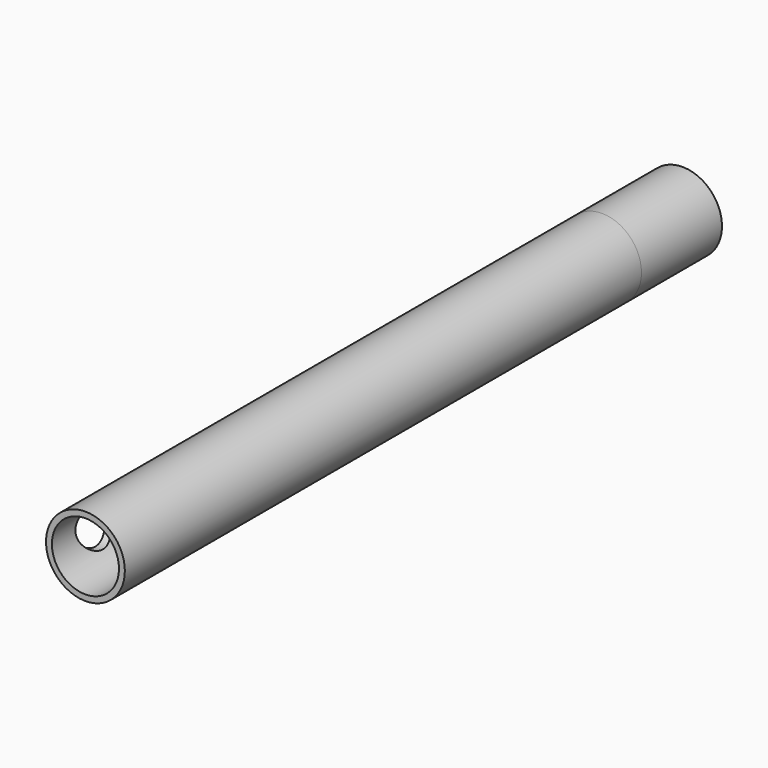
from build123d import *

# Parameters (mm, degrees)
F3_R      = 4.7
F4_DEPTH  = 67
F8_DEPTH  = 67
F6_R      = 4.7
F6_R_2    = 4
F9_DEPTH  = 10
F7_R      = 4.7
F7_R_2    = 4
F10_DEPTH = 12
F11_R     = 2.75
F12_DEPTH = 4.701


# Not quite as in the source:
# - ends of sketch curves that miss each other by under 0.0002 mm in the source are joined


with BuildPart() as f4:
    # F3 (on Front) → F4 (new body)
    with BuildSketch(Plane.XZ):
        Circle(F3_R)
    extrude(amount=F4_DEPTH)

    # F5 (on face) → F8 (cut, through all)
    with BuildSketch(Plane.XZ.offset(67)):
        with BuildLine():
            Line((-1.25, -3.8), (0, -3.8))
            Line((0, -3.8), (1.25, -3.8))
            Line((1.25, -3.8), (1.25, -3.7))
            ThreePointArc((1.25, -3.7), (1.3085786438, -3.5585786438), (1.45, -3.5))
            Line((1.45, -3.5), (2, -3.5))
            Line((2, -3.5), (2, -3.05))
            ThreePointArc((2, -3.05), (2.0585786438, -2.9085786438), (2.2, -2.85))
            Line((2.2, -2.85), (3.15, -2.85))
            Line((3.15, -2.85), (3.15, -2.15))
            Line((3.15, -2.15), (2.2, -2.15))
            ThreePointArc((2.2, -2.15), (2.0585786438, -2.0914213562), (2, -1.95))
            Line((2, -1.95), (2, -1.887459))
            ThreePointArc((2, -1.887459), (2.1033535752, -1.771554046), (2.2, -1.65))
            Line((2.2, -1.65), (3.75, -1.65))
            Line((3.75, -1.65), (3.75, 0))
            Line((3.75, 0), (3.75, 1.65))
            Line((3.75, 1.65), (2.2, 1.65))
            ThreePointArc((2.2, 1.65), (2.1033535752, 1.771554046), (1.9999998047, 1.8874588157))
            Line((1.9999998047, 1.8874588157), (2, 1.95))
            ThreePointArc((2, 1.95), (2.0585786438, 2.0914213562), (2.2, 2.15))
            Line((2.2, 2.15), (3.15, 2.15))
            Line((3.15, 2.15), (3.15, 2.85))
            Line((3.15, 2.85), (2.2, 2.85))
            ThreePointArc((2.2, 2.85), (2.0585786438, 2.9085786438), (2, 3.05))
            Line((2, 3.05), (2, 3.5))
            Line((2, 3.5), (1.45, 3.5))
            ThreePointArc((1.45, 3.5), (1.3085786438, 3.5585786438), (1.25, 3.7))
            Line((1.25, 3.7), (1.25, 3.8))
            Line((1.25, 3.8), (0, 3.8))
            Line((0, 3.8), (-1.25, 3.8))
            Line((-1.25, 3.8), (-1.25, 3.7))
            ThreePointArc((-1.25, 3.7), (-1.3085786438, 3.5585786438), (-1.45, 3.5))
            Line((-1.45, 3.5), (-2, 3.5))
            Line((-2, 3.5), (-2, 3.05))
            ThreePointArc((-2, 3.05), (-2.0585786438, 2.9085786438), (-2.2, 2.85))
            Line((-2.2, 2.85), (-3.15, 2.85))
            Line((-3.15, 2.85), (-3.15, 2.15))
            Line((-3.15, 2.15), (-2.2, 2.15))
            ThreePointArc((-2.2, 2.15), (-2.0585786438, 2.0914213562), (-2, 1.95))
            Line((-2, 1.95), (-2, 1.887459))
            ThreePointArc((-2, 1.887459), (-2.1033535752, 1.771554046), (-2.2, 1.65))
            Line((-2.2, 1.65), (-3.75, 1.65))
            Line((-3.75, 1.65), (-3.75, 0))
            Line((-3.75, 0), (-3.75, -1.65))
            Line((-3.75, -1.65), (-2.2, -1.65))
            ThreePointArc((-2.2, -1.65), (-2.1033535752, -1.771554046), (-1.9999998047, -1.8874588157))
            Line((-1.9999998047, -1.8874588157), (-2, -1.95))
            ThreePointArc((-2, -1.95), (-2.0585786438, -2.0914213562), (-2.2, -2.15))
            Line((-2.2, -2.15), (-3.15, -2.15))
            Line((-3.15, -2.15), (-3.15, -2.85))
            Line((-3.15, -2.85), (-2.2, -2.85))
            ThreePointArc((-2.2, -2.85), (-2.0585786438, -2.9085786438), (-2, -3.05))
            Line((-2, -3.05), (-2, -3.5))
            Line((-2, -3.5), (-1.45, -3.5))
            ThreePointArc((-1.45, -3.5), (-1.3085786438, -3.5585786438), (-1.25, -3.7))
            Line((-1.25, -3.7), (-1.25, -3.8))
        make_face()
    extrude(amount=-F8_DEPTH, mode=Mode.SUBTRACT)

    # F6 (on face) → F9 (join)
    with BuildSketch(Plane.XZ.offset(67)):
        Circle(F6_R)
        Circle(F6_R_2, mode=Mode.SUBTRACT)
    extrude(amount=F9_DEPTH)

    # F7 (on face) → F10 (join)
    with BuildSketch(Plane(origin=(0, 0, 0), x_dir=(-1, 0, 0), z_dir=(0, 1, 0))):
        Circle(F7_R)
        Circle(F7_R_2, mode=Mode.SUBTRACT)
    extrude(amount=F10_DEPTH)

    # F11 (on Right) → F12 (cut, through all)
    with BuildSketch(Plane.YZ):
        with Locations((-70.75, 0)):
            Circle(F11_R)
    extrude(amount=-F12_DEPTH, mode=Mode.SUBTRACT)


solid = f4.part
